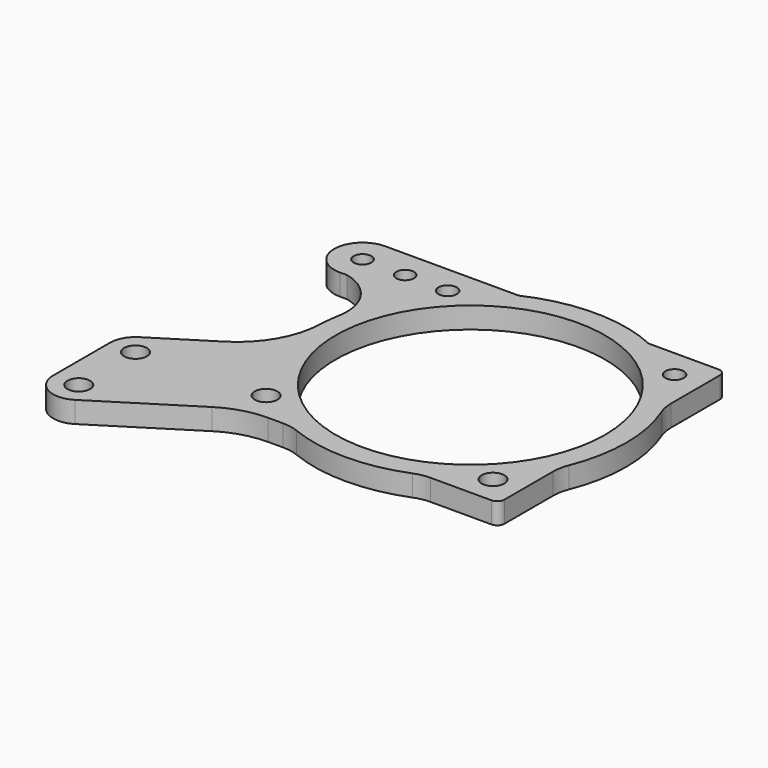
from build123d import *

# Parameters (mm, degrees)
F0_R     = 1.6
F0_R_2   = 1.25
F0_R_3   = 1.3
F0_R_4   = 19
F1_DEPTH = 3


# Not quite as in the source:
# - ends of sketch curves that miss each other by under 0.0002 mm in the source are joined


with BuildPart() as f1:
    # F0 (on Top) → F1 (new body)
    with BuildSketch(Plane.XY):
        with BuildLine():
            ThreePointArc((26.65, -15.75), (27.3571067812, -15.4571067812), (27.65, -14.75))
            Line((27.65, -14.75), (27.65, -6.142305))
            ThreePointArc((27.65, -6.142305), (27.7581169954, -5.008411416), (28.0785715533, -3.9153822211))
            ThreePointArc((28.0785715533, -3.9153822211), (29.65, 4.25), (28.0785715, 12.4153821998))
            ThreePointArc((28.0785715, 12.4153821998), (27.7581169954, 13.508411416), (27.65, 14.642305))
            Line((27.65, 14.642305), (27.65, 23.25))
            ThreePointArc((27.65, 23.25), (27.3571067812, 23.9571067812), (26.65, 24.25))
            Line((26.65, 24.25), (16.815151, 24.25))
            ThreePointArc((16.815151, 24.25), (7.65, 26.25), (-1.5151510677, 24.2500001477))
            Line((-1.5151510677, 24.2500001477), (-20.35, 24.25))
            ThreePointArc((-20.35, 24.25), (-24.35, 20.25), (-20.35, 16.25))
            Line((-20.35, 16.25), (-19.325715, 16.25))
            ThreePointArc((-19.325715, 16.25), (-15.0422529035, 13.2818239509), (-13.9967824398, 8.1764238984))
            ThreePointArc((-13.9967824398, 8.1764238984), (-14.2174174888, 6.6616493047), (-14.3321842117, 5.1351990085))
            ThreePointArc((-14.3321842117, 5.1351990085), (-15.9346176497, -0.3896755352), (-19.9242382655, -4.5339435787))
            Line((-19.9242382655, -4.5339435787), (-27.969469, -9.604406))
            ThreePointArc((-27.969469, -9.604406), (-29.2019904282, -10.9107598382), (-29.65, -12.65))
            Line((-29.65, -12.65), (-29.65, -22.65))
            ThreePointArc((-29.65, -22.65), (-27.7892401618, -25.8019904282), (-24.1305313003, -25.6955935236))
            Line((-24.1305313003, -25.6955935236), (-11.282229, -17.598022))
            ThreePointArc((-11.282229, -17.598022), (-8.2138844175, -16.2212589687), (-4.884, -15.75))
            Line((-4.884, -15.75), (-2.742305, -15.75))
            ThreePointArc((-2.742305, -15.75), (-1.608411416, -15.8581169954), (-0.5153822211, -16.1785715533))
            ThreePointArc((-0.5153822211, -16.1785715533), (7.65, -17.75), (15.8153821998, -16.1785715))
            ThreePointArc((15.8153821998, -16.1785715), (16.908411416, -15.8581169954), (18.042305, -15.75))
            Line((18.042305, -15.75), (26.65, -15.75))
        make_face()
        with Locations((-26.05, -22.65)):
            Circle(F0_R, mode=Mode.SUBTRACT)
        with Locations((-26.05, -12.65)):
            Circle(F0_R, mode=Mode.SUBTRACT)
        with Locations((-8.35, -11.75)):
            Circle(F0_R, mode=Mode.SUBTRACT)
        with Locations((23.65, -11.75)):
            Circle(F0_R, mode=Mode.SUBTRACT)
        with Locations((-20.35, 20.25)):
            Circle(F0_R_2, mode=Mode.SUBTRACT)
        with Locations((-14.35, 20.25)):
            Circle(F0_R_2, mode=Mode.SUBTRACT)
        with Locations((-8.35, 20.25)):
            Circle(F0_R_3, mode=Mode.SUBTRACT)
        with Locations((7.65, 4.25)):
            Circle(F0_R_4, mode=Mode.SUBTRACT)
        with Locations((23.65, 20.25)):
            Circle(F0_R_3, mode=Mode.SUBTRACT)
    extrude(amount=F1_DEPTH)


solid = f1.part
